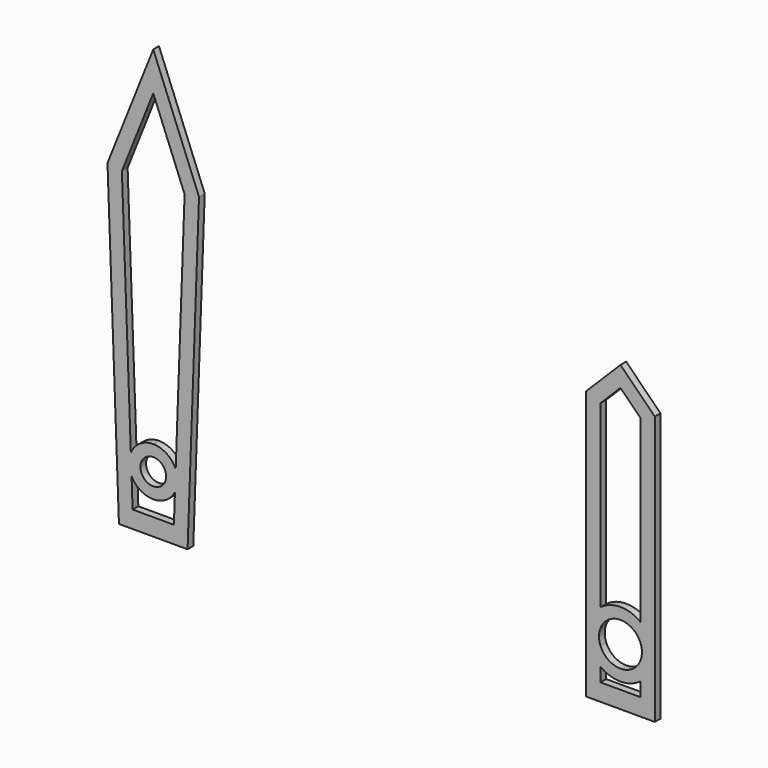
from build123d import *

# Parameters (mm, degrees)
F1_DEPTH = 0.25
F0_W     = 3
F0_H     = 0.6


# Not quite as in the source:
# - a feature names something its author has since deleted; it is built from what else it names


with BuildPart() as f1:
    # F0 (on Front) → F1 (new body)
    with BuildSketch(Plane.XZ):
        with BuildLine():
            Line((-21.4497518182, 1.5), (-21.4497518182, 0))
            Line((-21.4497518182, 0), (-21.3997518182, 0))
            ThreePointArc((-21.3997518182, 0), (-21.2811343854, 0.5086747487), (-20.9497518182, 0.9124143795))
            Line((-20.9497518182, 0.9124143795), (-20.9497518182, 1.5))
            Line((-20.9497518182, 1.5), (-20.9497518182, 7.1928932188))
            Line((-20.9497518182, 7.1928932188), (-20.2497518182, 7.8928932188))
            Line((-20.2497518182, 7.8928932188), (-19.5497518182, 7.1928932188))
            Line((-19.5497518182, 7.1928932188), (-19.5497518182, 1.5))
            Line((-19.5497518182, 1.5), (-19.5497518182, 0.9124143795))
            ThreePointArc((-19.5497518182, 0.9124143795), (-19.2183692509, 0.5086747487), (-19.0997518182, 0))
            ThreePointArc((-19.0997518182, 0), (-19.2183692509, -0.5086747487), (-19.5497518182, -0.9124143795))
            Line((-19.5497518182, -0.9124143795), (-19.5497518182, -1.4))
            Line((-19.5497518182, -1.4), (-19.0497518182, -1.4))
            Line((-19.0497518182, -1.4), (-19.0497518182, 1.5))
            Line((-19.0497518182, 1.5), (-19.0497518182, 7.4))
            Line((-19.0497518182, 7.4), (-20.2497518182, 8.6))
            Line((-20.2497518182, 8.6), (-21.4497518182, 7.4))
            Line((-21.4497518182, 7.4), (-21.4497518182, 1.5))
        make_face()
        with BuildLine():
            Line((-21.3997518182, 0), (-21.4497518182, 0))
            Line((-21.4497518182, 0), (-21.4497518182, -1.4))
            Line((-21.4497518182, -1.4), (-20.9497518182, -1.4))
            Line((-20.9497518182, -1.4), (-20.9497518182, -0.9124143795))
            ThreePointArc((-20.9497518182, -0.9124143795), (-21.2811343854, -0.5086747487), (-21.3997518182, 0))
        make_face()
        Polygon((-20.9497518182, -1.4), (-21.4497518182, -1.4), (-21.4497518182, -2), (-20.2497518182, -2), (-19.0497518182, -2), (-19.0497518182, -1.4), (-19.5497518182, -1.4), (-20.2497518182, -1.4), align=None)
        with BuildLine():
            ThreePointArc((-19.5497518182, 0.9124143795), (-20.2497518182, 1.15), (-20.9497518182, 0.9124143795))
            Line((-20.9497518182, 0.9124143795), (-20.9497518182, 0.2692582404))
            ThreePointArc((-20.9497518182, 0.2692582404), (-20.2497518182, 0.75), (-19.5497518182, 0.2692582404))
            Line((-19.5497518182, 0.2692582404), (-19.5497518182, 0.9124143795))
        make_face()
        with BuildLine():
            ThreePointArc((-19.0997518182, 0), (-19.2183692509, 0.5086747487), (-19.5497518182, 0.9124143795))
            Line((-19.5497518182, 0.9124143795), (-19.5497518182, 0.2692582404))
            ThreePointArc((-19.5497518182, 0.2692582404), (-19.512357758, 0.1369306394), (-19.4997518182, 0))
            ThreePointArc((-19.4997518182, 0), (-19.512357758, -0.1369306394), (-19.5497518182, -0.2692582404))
            Line((-19.5497518182, -0.2692582404), (-19.5497518182, -0.9124143795))
            ThreePointArc((-19.5497518182, -0.9124143795), (-19.2183692509, -0.5086747487), (-19.0997518182, 0))
        make_face()
        with BuildLine():
            Line((-20.9497518182, -0.2692582404), (-20.9497518182, -0.9124143795))
            ThreePointArc((-20.9497518182, -0.9124143795), (-20.2497518182, -1.15), (-19.5497518182, -0.9124143795))
            Line((-19.5497518182, -0.9124143795), (-19.5497518182, -0.2692582404))
            ThreePointArc((-19.5497518182, -0.2692582404), (-20.2497518182, -0.75), (-20.9497518182, -0.2692582404))
        make_face()
        with BuildLine():
            Line((-20.9997518182, 0), (-21.3997518182, 0))
            ThreePointArc((-21.3997518182, 0), (-21.2811343854, -0.5086747487), (-20.9497518182, -0.9124143795))
            Line((-20.9497518182, -0.9124143795), (-20.9497518182, -0.2692582404))
            ThreePointArc((-20.9497518182, -0.2692582404), (-20.9871458784, -0.1369306394), (-20.9997518182, 0))
        make_face()
        with BuildLine():
            ThreePointArc((-20.9497518182, 0.9124143795), (-21.2811343854, 0.5086747487), (-21.3997518182, 0))
            Line((-21.3997518182, 0), (-20.9997518182, 0))
            ThreePointArc((-20.9997518182, 0), (-20.9871458784, 0.1369306394), (-20.9497518182, 0.2692582404))
            Line((-20.9497518182, 0.2692582404), (-20.9497518182, 0.9124143795))
        make_face()
    extrude(amount=F1_DEPTH)


with BuildPart() as f1b:
    # F0 (on Front) → F1, piece 2 (new body)
    with BuildSketch(Plane.XZ):
        with BuildLine():
            ThreePointArc((-28.7187018186, 0.6873863542), (-29.0461968385, 0.4107919181), (-29.1687018186, 0))
            Line((-29.1687018186, 0), (-28.7687018186, 0))
            ThreePointArc((-28.7687018186, 0), (-28.7559702577, 0.0935414347), (-28.7187018186, 0.1802775638))
            Line((-28.7187018186, 0.1802775638), (-28.7187018186, 0.6873863542))
        make_face()
        with BuildLine():
            Line((-28.7687018186, 0), (-29.1687018186, 0))
            ThreePointArc((-29.1687018186, 0), (-29.0461968385, -0.4107919181), (-28.7187018186, -0.6873863542))
            Line((-28.7187018186, -0.6873863542), (-28.7187018186, -0.1802775638))
            ThreePointArc((-28.7187018186, -0.1802775638), (-28.7559702577, -0.0935414347), (-28.7687018186, 0))
        make_face()
        with BuildLine():
            Line((-28.7187018186, 12.9938064694), (-28.7187018186, 0.6873863542))
            ThreePointArc((-28.7187018186, 0.6873863542), (-28.5719340514, 0.7341797347), (-28.4187018186, 0.75))
            Line((-28.4187018186, 0.75), (-28.4187018186, 12.9938064694))
            Line((-28.4187018186, 12.9938064694), (-28.7187018186, 12.9938064694))
        make_face()
        with BuildLine():
            ThreePointArc((-28.4187018186, 0.75), (-28.5719340514, 0.7341797347), (-28.7187018186, 0.6873863542))
            Line((-28.7187018186, 0.6873863542), (-28.7187018186, 0.1802775638))
            ThreePointArc((-28.7187018186, 0.1802775638), (-28.5910428362, 0.3046285831), (-28.4187018186, 0.35))
            Line((-28.4187018186, 0.35), (-28.4187018186, 0.75))
        make_face()
        with BuildLine():
            Line((-28.7187018186, -0.1802775638), (-28.7187018186, -0.6873863542))
            ThreePointArc((-28.7187018186, -0.6873863542), (-28.5719340514, -0.7341797347), (-28.4187018186, -0.75))
            Line((-28.4187018186, -0.75), (-28.4187018186, -0.35))
            ThreePointArc((-28.4187018186, -0.35), (-28.5910428362, -0.3046285831), (-28.7187018186, -0.1802775638))
        make_face()
        with BuildLine():
            ThreePointArc((-28.4187018186, -0.75), (-28.5719340514, -0.7341797347), (-28.7187018186, -0.6873863542))
            Line((-28.7187018186, -0.6873863542), (-28.7187018186, -12.9938064694))
            Line((-28.7187018186, -12.9938064694), (-28.4187018186, -12.9938064694))
            Line((-28.4187018186, -12.9938064694), (-28.4187018186, -0.75))
        make_face()
        with BuildLine():
            Line((-28.4187018186, 12.9938064694), (-28.4187018186, 0.75))
            ThreePointArc((-28.4187018186, 0.75), (-28.2654695858, 0.7341797347), (-28.1187018186, 0.6873863542))
            Line((-28.1187018186, 0.6873863542), (-28.1187018186, 12.9938064694))
            Line((-28.1187018186, 12.9938064694), (-28.4187018186, 12.9938064694))
        make_face()
        with BuildLine():
            ThreePointArc((-28.1187018186, 0.6873863542), (-28.2654695858, 0.7341797347), (-28.4187018186, 0.75))
            Line((-28.4187018186, 0.75), (-28.4187018186, 0.35))
            ThreePointArc((-28.4187018186, 0.35), (-28.246360801, 0.3046285831), (-28.1187018186, 0.1802775638))
            Line((-28.1187018186, 0.1802775638), (-28.1187018186, 0.6873863542))
        make_face()
        with BuildLine():
            Line((-28.4187018186, -0.35), (-28.4187018186, -0.75))
            ThreePointArc((-28.4187018186, -0.75), (-28.2654695858, -0.7341797347), (-28.1187018186, -0.6873863542))
            Line((-28.1187018186, -0.6873863542), (-28.1187018186, -0.1802775638))
            ThreePointArc((-28.1187018186, -0.1802775638), (-28.246360801, -0.3046285831), (-28.4187018186, -0.35))
        make_face()
        with BuildLine():
            ThreePointArc((-28.1187018186, -0.6873863542), (-28.2654695858, -0.7341797347), (-28.4187018186, -0.75))
            Line((-28.4187018186, -0.75), (-28.4187018186, -12.9938064694))
            Line((-28.4187018186, -12.9938064694), (-28.1187018186, -12.9938064694))
            Line((-28.1187018186, -12.9938064694), (-28.1187018186, -0.6873863542))
        make_face()
        with BuildLine():
            ThreePointArc((-27.6687018186, 0), (-27.7912067987, 0.4107919181), (-28.1187018186, 0.6873863542))
            Line((-28.1187018186, 0.6873863542), (-28.1187018186, 0.1802775638))
            ThreePointArc((-28.1187018186, 0.1802775638), (-28.0814333795, 0.0935414347), (-28.0687018186, 0))
            Line((-28.0687018186, 0), (-27.6687018186, 0))
        make_face()
        with BuildLine():
            Line((-28.1187018186, -0.1802775638), (-28.1187018186, -0.6873863542))
            ThreePointArc((-28.1187018186, -0.6873863542), (-27.7912067987, -0.4107919181), (-27.6687018186, 0))
            Line((-27.6687018186, 0), (-28.0687018186, 0))
            ThreePointArc((-28.0687018186, 0), (-28.0814333795, -0.0935414347), (-28.1187018186, -0.1802775638))
        make_face()
    extrude(amount=F1_DEPTH)


with BuildPart() as f1c:
    # F0 (on Front) → F1, piece 3 (new body)
    with BuildSketch(Plane.XZ):
        with BuildLine():
            Line((-34.987651819, 8.9829219505), (-36.587651819, 13))
            Line((-36.587651819, 13), (-36.587651819, 11.6487521661))
            Line((-36.587651819, 11.6487521661), (-35.4911559916, 8.8958088415))
            Line((-35.4911559916, 8.8958088415), (-35.8032202993, 0.3273640038))
            ThreePointArc((-35.8032202993, 0.3273640038), (-35.7542051225, 0.1669329331), (-35.737651819, 0))
            Line((-35.737651819, 0), (-35.314811458, 0))
            Line((-35.314811458, 0), (-34.987651819, 8.9829219505))
        make_face()
        with BuildLine():
            Line((-36.587651819, 11.6487521661), (-36.587651819, 13))
            Line((-36.587651819, 13), (-38.187651819, 8.9829219505))
            Line((-38.187651819, 8.9829219505), (-37.787651819, -2))
            Line((-37.787651819, -2), (-36.587651819, -2))
            Line((-36.587651819, -2), (-35.387651819, -2))
            Line((-35.387651819, -2), (-35.314811458, 0))
            Line((-35.314811458, 0), (-35.737651819, 0))
            ThreePointArc((-35.737651819, 0), (-35.7608330268, -0.1971564985), (-35.829112254, -0.3835592892))
            Line((-35.829112254, -0.3835592892), (-35.8661312082, -1.4))
            Line((-35.8661312082, -1.4), (-36.587651819, -1.4))
            Line((-36.587651819, -1.4), (-37.3091724298, -1.4))
            Line((-37.3091724298, -1.4), (-37.346191384, -0.3835592892))
            ThreePointArc((-37.346191384, -0.3835592892), (-37.4370886466, -0.0309366426), (-37.3720833386, 0.3273640038))
            Line((-37.3720833386, 0.3273640038), (-37.6841476463, 8.8958088415))
            Line((-37.6841476463, 8.8958088415), (-36.587651819, 11.6487521661))
        make_face()
        with BuildLine():
            ThreePointArc((-35.829112254, -0.3835592892), (-35.7608330268, -0.1971564985), (-35.737651819, 0))
            Line((-35.737651819, 0), (-36.137651819, 0))
            ThreePointArc((-36.137651819, 0), (-36.9058498705, -0.3181980515), (-36.587651819, 0.45))
            Line((-36.587651819, 0.45), (-36.587651819, 0.85))
            ThreePointArc((-36.587651819, 0.85), (-37.0589482208, 0.7073752198), (-37.3720833386, 0.3273640038))
            ThreePointArc((-37.3720833386, 0.3273640038), (-37.4370886466, -0.0309366426), (-37.346191384, -0.3835592892))
            ThreePointArc((-37.346191384, -0.3835592892), (-36.587651819, -0.85), (-35.829112254, -0.3835592892))
        make_face()
        with BuildLine():
            Line((-36.137651819, 0), (-35.737651819, 0))
            ThreePointArc((-35.737651819, 0), (-35.7542051225, 0.1669329331), (-35.8032202993, 0.3273640038))
            ThreePointArc((-35.8032202993, 0.3273640038), (-36.1163554172, 0.7073752198), (-36.587651819, 0.85))
            Line((-36.587651819, 0.85), (-36.587651819, 0.45))
            ThreePointArc((-36.587651819, 0.45), (-36.2694537675, 0.3181980515), (-36.137651819, 0))
        make_face()
    extrude(amount=F1_DEPTH)


with BuildPart() as f1d:
    # F0 (on Front) → F1, piece 4 (new body)
    with BuildSketch(Plane.XZ):
        with Locations((-24.663922295, 11.3997036099)):
            Rectangle(F0_W, F0_H)
    extrude(amount=F1_DEPTH)


with BuildPart() as f1e:
    # F0 (on Front) → F1, piece 5 (new body)
    with BuildSketch(Plane.XZ):
        with Locations((-24.663922295, 9.8090009272)):
            Rectangle(F0_W, F0_H)
    extrude(amount=F1_DEPTH)


solid = Compound([f1.part, f1c.part])
